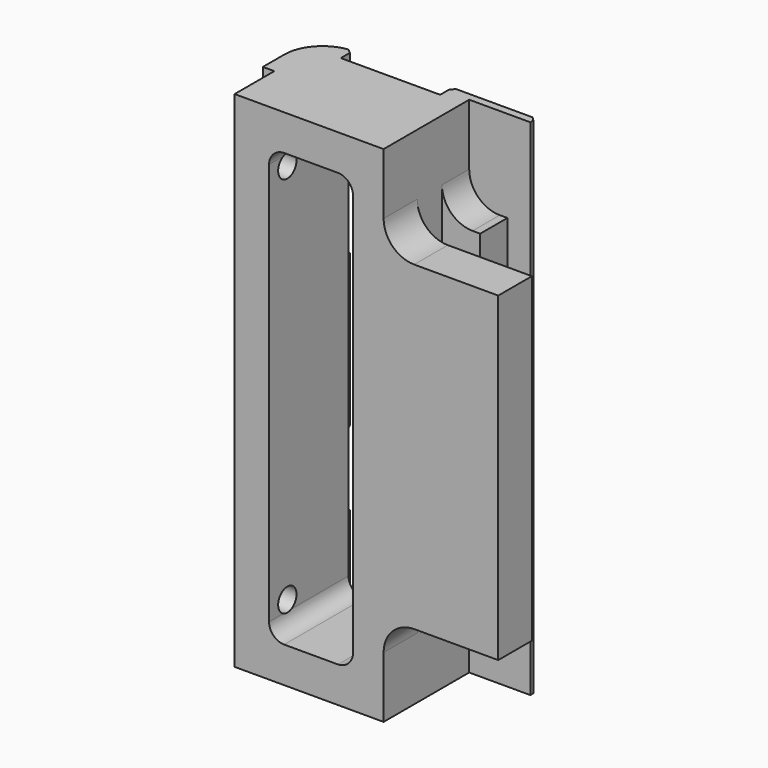
from build123d import *

# Parameters (mm, degrees)
F0_W           = 21
F0_H           = 66
F0_W_2         = 11
F0_H_2         = 56.642
F1_DEPTH       = 15
F2_R           = 5
F4_START       = 9.5
F3_W           = 15
F3_H           = 42
F4_DEPTH       = 5.5
F5_T1_DEPTH    = 15
F6_W           = 1.5
F6_H           = 6.5
F7_DEPTH       = 50
F7_DEPTH_BACK  = 50
F8_R           = 1.5
F9_DEPTH       = 5
F10_W          = 3
F10_H          = 1
F11_DEPTH      = 33
F11_DEPTH_BACK = 33
F12_SIZE       = 0.5
F13_W          = 5
F13_H          = 12
F14_DEPTH      = 14
F15_R          = 4
F16_W          = 13
F16_H          = 70
F17_DEPTH      = 2
F18_W          = 20
F18_H          = 12
F19_DEPTH      = 2
F20_R          = 2
F21_T1_DEPTH   = 68.8536746712
F21_T3_DEPTH   = 11.490341494
F21_T5_DEPTH   = 3
F21_T7_DEPTH   = 8
F21_T9_DEPTH   = 11.490341494
F21_T11_DEPTH  = 13.591
F21_T13_DEPTH  = 8
F21_T16_ANGLE  = 90
F21_T18_ANGLE  = 90
F21_T20_ANGLE  = 90
F21_T22_ANGLE  = 90
F21_T24_ANGLE  = 90
F21_T26_ANGLE  = 90
F21_T28_ANGLE  = 90
F21_T30_ANGLE  = 90
F23_START      = -6.5
F22_R          = 6
F23_DEPTH      = 5.001


# Not quite as in the source:
# - a fillet or chamfer that OpenCascade refuses, or shapes differently, is made with other operations: its cross-section is extruded or revolved along the edge and cut away or added


with BuildPart() as f1:
    # F0 (on Front) → F1 (new body)
    with BuildSketch(Plane.XZ):
        with Locations((-1, 0)):
            Rectangle(F0_W, F0_H)
        Rectangle(F0_W_2, F0_H_2, mode=Mode.SUBTRACT)
    extrude(amount=F1_DEPTH)

    # F2
    f2_edges = [f1.edges().sort_by_distance(p)[0] for p in [
        (-11.5, 0, 0),
    ]]
    fillet(f2_edges, radius=F2_R)

    # F3 (on Front) → F4 (join)
    with BuildSketch(Plane.XZ.offset(F4_START)):
        with Locations((17, 0)):
            Rectangle(F3_W, F3_H)
    extrude(amount=F4_DEPTH)

    # F5: fillet of radius 2 on 4 edges, made by hand

    # F5_s2 → F5_t1 (join)
    with BuildSketch(Plane.XZ):
        with BuildLine():
            ThreePointArc((5.5001, -26.3211), (4.9143135624, -27.7353135624), (3.5001, -28.3211))
            Line((3.5001, -28.3211), (3.5001, -28.3611))
            ThreePointArc((3.5001, -28.3611), (4.50005, -28.361), (5.5, -28.361))
            Line((5.5, -28.361), (5.54, -28.321))
            ThreePointArc((5.54, -28.321), (5.54, -27.32105), (5.5401, -26.3211))
            Line((5.5401, -26.3211), (5.5001, -26.3211))
        make_face()
        with BuildLine():
            ThreePointArc((-3.5001, -28.3211), (-4.9143135624, -27.7353135624), (-5.5001, -26.3211))
            Line((-5.5001, -26.3211), (-5.5401, -26.3211))
            ThreePointArc((-5.5401, -26.3211), (-5.54, -27.32105), (-5.54, -28.321))
            Line((-5.54, -28.321), (-5.5, -28.361))
            ThreePointArc((-5.5, -28.361), (-4.50005, -28.361), (-3.5001, -28.3611))
            Line((-3.5001, -28.3611), (-3.5001, -28.3211))
        make_face()
        with BuildLine():
            ThreePointArc((-5.5001, 26.3211), (-4.9143135624, 27.7353135624), (-3.5001, 28.3211))
            Line((-3.5001, 28.3211), (-3.5001, 28.3611))
            ThreePointArc((-3.5001, 28.3611), (-4.50005, 28.361), (-5.5, 28.361))
            Line((-5.5, 28.361), (-5.54, 28.321))
            ThreePointArc((-5.54, 28.321), (-5.54, 27.32105), (-5.5401, 26.3211))
            Line((-5.5401, 26.3211), (-5.5001, 26.3211))
        make_face()
        with BuildLine():
            ThreePointArc((5.5001, 26.3211), (4.9143135624, 27.7353135624), (3.5001, 28.3211))
            Line((3.5001, 28.3211), (3.5001, 28.3611))
            ThreePointArc((3.5001, 28.3611), (4.50005, 28.361), (5.5, 28.361))
            Line((5.5, 28.361), (5.54, 28.321))
            ThreePointArc((5.54, 28.321), (5.54, 27.32105), (5.5401, 26.3211))
            Line((5.5401, 26.3211), (5.5001, 26.3211))
        make_face()
    extrude(amount=F5_T1_DEPTH)

    # F6 (on Top) → F7 (cut, two sides)
    with BuildSketch(Plane.XY) as f7_sk:
        with Locations((-10.75, -11.75)):
            Rectangle(F6_W, F6_H)
    extrude(amount=-F7_DEPTH, mode=Mode.SUBTRACT)
    extrude(f7_sk.sketch, amount=F7_DEPTH_BACK, mode=Mode.SUBTRACT)

    # F8 (on face) → F9 (cut)
    with BuildSketch(Plane(origin=(-10, 0, 0), x_dir=(0, -1, 0), z_dir=(-1, 0, 0))):
        with Locations((12, 25)):
            Circle(F8_R)
        with Locations((12, -25)):
            Circle(F8_R)
    extrude(amount=-F9_DEPTH, mode=Mode.SUBTRACT)

    # F10 (on Top) → F11 (join, two sides)
    with BuildSketch(Plane.XY) as f11_sk:
        with Locations((16, -0.5)):
            Rectangle(F10_W, F10_H)
        Polygon((14.5, -5.45), (14.5, -1), (14.5, 0), (9.5, 0), (9.5, -5.45), align=None)
    extrude(amount=F11_DEPTH)
    extrude(f11_sk.sketch, amount=-F11_DEPTH_BACK)

    # F12
    f12_edges = [f1.edges().sort_by_distance(p)[0] for p in [
        (17.5, 0, 0),
    ]]
    chamfer(f12_edges, length=F12_SIZE)

    # F13 (on face) → F14 (cut)
    with BuildSketch(Plane.XZ.offset(15)):
        with Locations((12, -27)):
            Rectangle(F13_W, F13_H)
        with Locations((12, 27)):
            Rectangle(F13_W, F13_H)
    extrude(amount=-F14_DEPTH, mode=Mode.SUBTRACT)

    # F15
    f15_edges = [f1.edges().sort_by_distance(p)[0] for p in [
        (9.5, -3.225, -21),
        (9.5, -12.25, -21),
        (9.5, -3.225, 21),
        (9.5, -12.25, 21),
    ]]
    fillet(f15_edges, radius=F15_R)

    # F16 (on Front) → F17 (cut)
    with BuildSketch(Plane.XZ):
        Rectangle(F16_W, F16_H)
    extrude(amount=F17_DEPTH, mode=Mode.SUBTRACT)

    # F18 (on face) → F19 (cut)
    with BuildSketch(Plane(origin=(0, 0, 0), x_dir=(-1, 0, 0), z_dir=(0, 1, 0))):
        with Locations((-3.5, 14.7955)):
            Rectangle(F18_W, F18_H)
        with Locations((-3.5, -14.7955)):
            Rectangle(F18_W, F18_H)
    extrude(amount=-F19_DEPTH, mode=Mode.SUBTRACT)

    # F20
    f20_edges = [f1.edges().sort_by_distance(p)[0] for p in [
        (13.5, -1, -20.7955),
        (13.5, -1, 20.7955),
        (6.5, -1, 20.7955),
        (6.5, -1, 8.7955),
        (6.5, -1, -8.7955),
        (6.5, -1, -20.7955),
        (13.5, -1, -8.7955),
        (13.5, -1, 8.7955),
    ]]
    fillet(f20_edges, radius=F20_R)

    # F21: chamfer of 0.5 on 18 edges, made by hand

    # F21_s2 → F21_t1 (cut)
    with BuildSketch(Plane.XY.offset(-34.4268373356)):
        with BuildLine():
            Line((-7.0555555556, -0.03096005), (-6.5, -0.527864045))
            Line((-6.5, -0.527864045), (-6.5, 0))
            ThreePointArc((-6.5, 0), (-6.7852695606, -0.0081445055), (-7.0555555556, -0.03096005))
        make_face()
    extrude(amount=F21_T1_DEPTH, mode=Mode.SUBTRACT)

    # F21_s4 → F21_t3 (cut)
    with BuildSketch(Plane.XY.offset(-34.285841494)):
        Polygon((7, 0), (6.5, -0.5), (6.5, 0), align=None)
    extrude(amount=F21_T3_DEPTH, mode=Mode.SUBTRACT)

    # F21_s6 → F21_t5 (cut)
    with BuildSketch(Plane.YZ.offset(8.5)):
        Polygon((0, -21.2955), (-0.5, -20.7955), (0, -20.7955), align=None)
        Polygon((0, -8.2955), (-0.5, -8.7955), (0, -8.7955), align=None)
        Polygon((0, 21.2955), (-0.5, 20.7955), (0, 20.7955), align=None)
        Polygon((0, 8.2955), (-0.5, 8.7955), (0, 8.7955), align=None)
    extrude(amount=F21_T5_DEPTH, mode=Mode.SUBTRACT)

    # F21_s8 → F21_t7 (cut)
    with BuildSketch(Plane.XY.offset(-18.7955)):
        Polygon((14, 0), (13.5, -0.5), (13.5, 0), align=None)
    extrude(amount=F21_T7_DEPTH, mode=Mode.SUBTRACT)

    # F21_s10 → F21_t9 (cut)
    with BuildSketch(Plane.XY.offset(22.7955)):
        Polygon((7, 0), (6.5, -0.5), (6.5, 0), align=None)
    extrude(amount=F21_T9_DEPTH, mode=Mode.SUBTRACT)

    # F21_s12 → F21_t11 (cut)
    with BuildSketch(Plane.XY.offset(-6.7955)):
        Polygon((7, 0), (6.5, -0.5), (6.5, 0), align=None)
    extrude(amount=F21_T11_DEPTH, mode=Mode.SUBTRACT)

    # F21_s14 → F21_t13 (cut)
    with BuildSketch(Plane.XY.offset(10.7955)):
        Polygon((14, 0), (13.5, -0.5), (13.5, 0), align=None)
    extrude(amount=F21_T13_DEPTH, mode=Mode.SUBTRACT)

    # F21_s15 → F21_t16 (revolve, cut)
    with BuildSketch(Plane.YZ.offset(8.5)):
        Polygon((0, -21.2955), (-0.5, -20.7955), (0, -20.7955), align=None)
    revolve(axis=Axis((8.5, 0, -22.7955), (0, -1, 0)), revolution_arc=F21_T16_ANGLE, mode=Mode.SUBTRACT)

    # F21_s17 → F21_t18 (revolve, cut)
    with BuildSketch(Plane.XY.offset(-18.7955)):
        Polygon((14, 0), (13.5, -0.5), (13.5, 0), align=None)
    revolve(axis=Axis((11.5, 0, -18.7955), (0, 1, 0)), revolution_arc=F21_T18_ANGLE, mode=Mode.SUBTRACT)

    # F21_s19 → F21_t20 (revolve, cut)
    with BuildSketch(Plane.YZ.offset(11.5)):
        Polygon((0, -8.2955), (-0.5, -8.7955), (0, -8.7955), align=None)
    revolve(axis=Axis((11.5, 0, -10.7955), (0, 1, 0)), revolution_arc=F21_T20_ANGLE, mode=Mode.SUBTRACT)

    # F21_s21 → F21_t22 (revolve, cut)
    with BuildSketch(Plane.XY.offset(22.7955)):
        Polygon((7, 0), (6.5, -0.5), (6.5, 0), align=None)
    revolve(axis=Axis((8.5, 0, 22.7955), (0, -1, 0)), revolution_arc=F21_T22_ANGLE, mode=Mode.SUBTRACT)

    # F21_s23 → F21_t24 (revolve, cut)
    with BuildSketch(Plane.XY.offset(-6.7955)):
        Polygon((7, 0), (6.5, -0.5), (6.5, 0), align=None)
    revolve(axis=Axis((8.5, 0, -6.7955), (0, -1, 0)), revolution_arc=F21_T24_ANGLE, mode=Mode.SUBTRACT)

    # F21_s25 → F21_t26 (revolve, cut)
    with BuildSketch(Plane.YZ.offset(11.5)):
        Polygon((0, 21.2955), (-0.5, 20.7955), (0, 20.7955), align=None)
    revolve(axis=Axis((11.5, 0, 18.7955), (0, 1, 0)), revolution_arc=F21_T26_ANGLE, mode=Mode.SUBTRACT)

    # F21_s27 → F21_t28 (revolve, cut)
    with BuildSketch(Plane.YZ.offset(8.5)):
        Polygon((0, 8.2955), (-0.5, 8.7955), (0, 8.7955), align=None)
    revolve(axis=Axis((8.5, 0, 6.7955), (0, -1, 0)), revolution_arc=F21_T28_ANGLE, mode=Mode.SUBTRACT)

    # F21_s29 → F21_t30 (revolve, cut)
    with BuildSketch(Plane.XY.offset(10.7955)):
        Polygon((14, 0), (13.5, -0.5), (13.5, 0), align=None)
    revolve(axis=Axis((11.5, 0, 10.7955), (0, 1, 0)), revolution_arc=F21_T30_ANGLE, mode=Mode.SUBTRACT)

    # F22 (on Right) → F23 (cut)
    with BuildSketch(Plane.YZ.offset(F23_START)):
        with Locations((3, -14.7955)):
            Circle(F22_R)
        with Locations((3, 14.7955)):
            Circle(F22_R)
    extrude(amount=-F23_DEPTH, mode=Mode.SUBTRACT)


solid = f1.part
